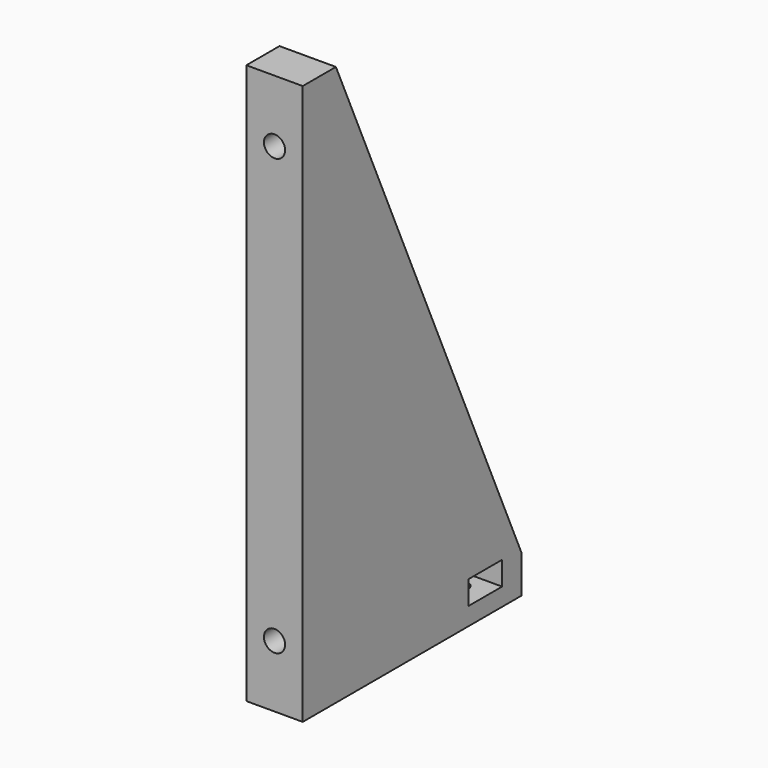
from build123d import *

# Parameters (mm, degrees)
F1_DEPTH  = 13.6
F3_D      = 5.1
F5_DEPTH  = 12
F6_DEPTH  = 25
F7_DEPTH  = 15
F8_D      = 5.1
F9_W      = 5.1
F9_H      = 5.7
F10_DEPTH = 25
F4_W      = 6.8
F4_H      = 4
F11_DEPTH = 25


# Not quite as in the source:
# - a feature names something its author has since deleted; it is built from what else it names


with BuildPart() as f1:
    # F0 (on Right) → F1 (new body)
    with BuildSketch(Plane.YZ):
        Polygon((-70, 0), (0, 0), (-60, 135), (-70, 135), align=None)
    extrude(amount=F1_DEPTH)

    # F3 (through all)
    with Locations(Plane.XZ.offset(70)):
        with Locations((6.8, 15), (6.8, 120)):
            Hole(F3_D / 2)

    # F4 (on face) → F5 (cut)
    with BuildSketch(Plane(origin=(0, 0, 0), x_dir=(1, 0, 0), z_dir=(0, 0, -1))):
        with BuildLine():
            ThreePointArc((9.35, 55), (8.603122292, 56.803122292), (6.8, 57.55))
            Line((6.8, 57.55), (6.8, 55))
            Line((6.8, 55), (6.8, 52.45))
            ThreePointArc((6.8, 52.45), (8.603122292, 53.196877708), (9.35, 55))
        make_face()
        with BuildLine():
            ThreePointArc((9.35, 15), (8.603122292, 16.803122292), (6.8, 17.55))
            ThreePointArc((6.8, 17.55), (4.996877708, 13.196877708), (9.35, 15))
        make_face()
        with BuildLine():
            Line((6.8, 55), (6.8, 57.55))
            ThreePointArc((6.8, 57.55), (4.25, 55), (6.8, 52.45))
            Line((6.8, 52.45), (6.8, 55))
        make_face()
    extrude(amount=-F5_DEPTH, mode=Mode.SUBTRACT)

    # F2 (on face) → F6 (join)
    with BuildSketch(Plane.XZ.offset(70)):
        Polygon((11.9, 122.9444863729), (6.8, 125.8889727457), (1.7, 122.9444863729), (1.7, 117.0555136271), (6.8, 114.1110272543), (11.9, 117.0555136271), align=None)
    extrude(amount=-F6_DEPTH)

    # F7 (cut): a face of the model
    f7_faces = [f1.faces().sort_by_distance(p)[0] for p in [
        (6.8, -45, 120),
    ]]
    extrude(f7_faces, amount=-F7_DEPTH, mode=Mode.SUBTRACT)

    # F8 (through all)
    with Locations(Plane.XZ.offset(70)):
        with Locations((6.8, 120)):
            Hole(F8_D / 2)

    # F9 (on face) → F10 (cut)
    with BuildSketch(Plane(origin=(0, 0, 0), x_dir=(0, -1, 0), z_dir=(-1, 0, 0))):
        with Locations((12.45, 7.15)):
            Rectangle(F9_W, F9_H)
        with Locations((17.55, 7.15)):
            Rectangle(F9_W, F9_H)
    extrude(amount=-F10_DEPTH, mode=Mode.SUBTRACT)

    # F4 (on face) → F11 (cut)
    with BuildSketch(Plane(origin=(0, 0, 0), x_dir=(1, 0, 0), z_dir=(0, 0, -1))):
        with Locations((10.2, 2)):
            Rectangle(F4_W, F4_H)
        with Locations((3.4, 2)):
            Rectangle(F4_W, F4_H)
    extrude(amount=-F11_DEPTH, mode=Mode.SUBTRACT)


solid = f1.part
